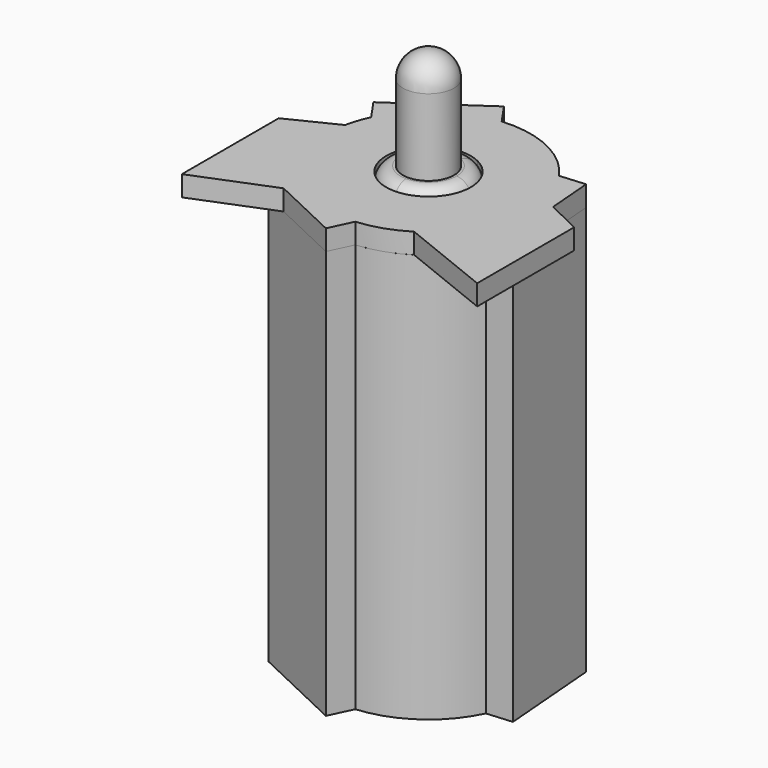
from build123d import *

# Parameters (mm, degrees)
F0_R     = 2.5
F1_DEPTH = 40
F2_DEPTH = 40
F3_R     = 2.5
F4_DEPTH = 10
F5_DEPTH = 2.5
F8_R     = 1.4
F9_DEPTH = 2


with BuildPart() as f1:
    # F0 (on Top) → F1 (new body)
    with BuildSketch(Plane.XY):
        with BuildLine():
            ThreePointArc((9.0374170739, -4.2807817782), (9.7563869014, -2.1938355979), (10, 0))
            ThreePointArc((10, 0), (9.5461967047, 2.9782760912), (8.2259743049, 5.6862418815))
            ThreePointArc((8.2259743049, 5.6862418815), (4.2807817782, 9.0374170739), (-0.8114427689, 9.9670236597))
            Line((-0.8114427689, 9.9670236597), (-9.0374170739, 4.2807817782))
            ThreePointArc((-9.0374170739, 4.2807817782), (-9.9670236597, -0.8114427689), (-8.2259743049, -5.6862418815))
            ThreePointArc((-8.2259743049, -5.6862418815), (-4.2807817782, -9.0374170739), (0.8114427689, -9.9670236597))
            ThreePointArc((0.8114427689, -9.9670236597), (5.6862418815, -8.2259743049), (9.0374170739, -4.2807817782))
        make_face()
        Circle(F0_R, mode=Mode.SUBTRACT)
        with BuildLine():
            ThreePointArc((8.2259743049, 5.6862418815), (9.5461967047, 2.9782760912), (10, 0))
            ThreePointArc((10, 0), (9.7563869014, -2.1938355979), (9.0374170739, -4.2807817782))
            Line((9.0374170739, -4.2807817782), (11.5291729888, -4.077921086))
            Line((11.5291729888, -4.077921086), (10.7177302199, 5.8891025737))
            Line((10.7177302199, 5.8891025737), (8.2259743049, 5.6862418815))
        make_face()
        with BuildLine():
            Line((-9.0374170739, 4.2807817782), (-0.8114427689, 9.9670236597))
            ThreePointArc((-0.8114427689, 9.9670236597), (-5.6862418815, 8.2259743049), (-9.0374170739, 4.2807817782))
        make_face()
        with BuildLine():
            ThreePointArc((-9.0374170739, 4.2807817782), (-5.6862418815, 8.2259743049), (-0.8114427689, 9.9670236597))
            Line((-0.8114427689, 9.9670236597), (-2.2330032393, 12.0235172359))
            Line((-2.2330032393, 12.0235172359), (-10.4589775442, 6.3372753545))
            Line((-10.4589775442, 6.3372753545), (-9.0374170739, 4.2807817782))
        make_face()
        with BuildLine():
            Line((-0.2587526756, -12.2263779282), (0.8114427689, -9.9670236597))
            ThreePointArc((0.8114427689, -9.9670236597), (-4.2807817782, -9.0374170739), (-8.2259743049, -5.6862418815))
            Line((-8.2259743049, -5.6862418815), (-9.2961697495, -7.9455961499))
            Line((-9.2961697495, -7.9455961499), (-0.2587526756, -12.2263779282))
        make_face()
    extrude(amount=F1_DEPTH)


with BuildPart() as f2:
    # F0 (on Top) → F2 (new body)
    with BuildSketch(Plane.XY):
        Circle(F0_R)
    extrude(amount=F2_DEPTH)

    # F3 (on face) → F4 (join)
    with BuildSketch(Plane.XY.offset(40)):
        Circle(F3_R)
    extrude(amount=F4_DEPTH)

    # F3 (on face) → F5 (join)
    with BuildSketch(Plane.XY.offset(40)):
        with BuildLine():
            ThreePointArc((1.8260342345, 3.7172857004), (-2.93e-08, 4.1415714414), (-1.8260342871, 3.7172856746))
            ThreePointArc((-1.8260342871, 3.7172856746), (-4.0341057369, -0.9373392702), (0, -4.1415714414))
            ThreePointArc((0, -4.1415714414), (2.928533251, -2.928533251), (4.1415714414, 0))
            ThreePointArc((4.1415714414, 0), (3.5153424613, 2.1897445933), (1.8260342345, 3.7172857004))
        make_face()
        Circle(F3_R, mode=Mode.SUBTRACT)
    extrude(amount=F5_DEPTH)

    # F6 (on Front) → F7 (revolve)
    with BuildSketch(Plane.XZ):
        with BuildLine():
            Line((-2.5, 50), (2.5, 50))
            ThreePointArc((2.5, 50), (0, 52.5), (-2.5, 50))
        make_face()
    revolve(axis=Axis((0, 0, 50), (-1, 0, 0)))

    # F8
    f8_edges = [f2.edges().sort_by_distance(p)[0] for p in [
        (1.826034, -3.717286, 42.5),
    ]]
    fillet(f8_edges, radius=F8_R)


with BuildPart() as f9:
    # F3 (on face) → F9 (new body)
    with BuildSketch(Plane.XY.offset(40)):
        with BuildLine():
            Line((11.2723216959, -0.9229938236), (1.8260342345, 3.7172857004))
            ThreePointArc((1.8260342345, 3.7172857004), (3.5153424613, 2.1897445933), (4.1415714414, 0))
            ThreePointArc((4.1415714414, 0), (2.928533251, -2.928533251), (0, -4.1415714414))
            Line((0, -4.1415714414), (7.1333343578, -7.008248065))
            ThreePointArc((7.1333343578, -7.008248065), (8.1995773399, -5.7242406874), (9.0374170739, -4.2807817782))
            Line((9.0374170739, -4.2807817782), (11.5291729888, -4.077921086))
            Line((11.5291729888, -4.077921086), (11.2723216959, -0.9229938236))
        make_face()
        with BuildLine():
            Line((1.8260342345, 3.7172857004), (0, 4.6142845799))
            Line((0, 4.6142845799), (-1.8260342871, 3.7172856746))
            ThreePointArc((-1.8260342871, 3.7172856746), (-2.93e-08, 4.1415714414), (1.8260342345, 3.7172857004))
        make_face()
        with BuildLine():
            ThreePointArc((-8.2259743049, -5.6862418815), (-9.5010919758, -3.1191747736), (-9.9956228645, -0.2958437956))
            Line((-9.9956228645, -0.2958437956), (-14.4493776544, -2.4836522061))
            Line((-14.4493776544, -2.4836522061), (-14.4493776544, -9.9483500207))
            Line((-14.4493776544, -9.9483500207), (-9.2562886562, -7.861400764))
            Line((-9.2562886562, -7.861400764), (-8.2259743049, -5.6862418815))
        make_face()
        with BuildLine():
            ThreePointArc((0, -4.1415714414), (-4.0341057369, -0.9373392702), (-1.8260342871, 3.7172856746))
            Line((-1.8260342871, 3.7172856746), (-9.9956228645, -0.2958437956))
            ThreePointArc((-9.9956228645, -0.2958437956), (-9.5010919758, -3.1191747736), (-8.2259743049, -5.6862418815))
            Line((-8.2259743049, -5.6862418815), (-9.2562886562, -7.861400764))
            Line((-9.2562886562, -7.861400764), (0, -4.1415714414))
        make_face()
        with BuildLine():
            Line((14.4493776544, -2.4836522061), (11.2723216959, -0.9229938236))
            Line((11.2723216959, -0.9229938236), (11.5291729888, -4.077921086))
            Line((11.5291729888, -4.077921086), (9.0374170739, -4.2807817782))
            ThreePointArc((9.0374170739, -4.2807817782), (8.1995773399, -5.7242406874), (7.1333343578, -7.008248065))
            Line((7.1333343578, -7.008248065), (14.4493776544, -9.9483500207))
            Line((14.4493776544, -9.9483500207), (14.4493776544, -2.4836522061))
        make_face()
        with BuildLine():
            Line((-14.4493776544, -2.4836522061), (-9.9956228645, -0.2958437956))
            ThreePointArc((-9.9956228645, -0.2958437956), (-9.9616891791, 0.8744991134), (-9.7911952771, 2.0328539162))
            Line((-9.7911952771, 2.0328539162), (-14.4493776544, -0.2553750195))
            Line((-14.4493776544, -0.2553750195), (-14.4493776544, -2.4836522061))
        make_face()
        Polygon((11.0833543073, 1.398109408), (11.2723216959, -0.9229938236), (14.4493776544, -2.4836522061), (14.4493776544, -0.2553750195), align=None)
        with BuildLine():
            Line((14.4493776544, -9.9483500207), (7.1333343578, -7.008248065))
            ThreePointArc((7.1333343578, -7.008248065), (6.2837328899, -7.7791195497), (5.3514333814, -8.4476127258))
            Line((5.3514333814, -8.4476127258), (14.4493776544, -12.1038081124))
            Line((14.4493776544, -12.1038081124), (14.4493776544, -9.9483500207))
        make_face()
        Polygon((-9.2961697495, -7.9455961499), (-9.2562886562, -7.861400764), (-14.4493776544, -9.9483500207), (-14.4493776544, -12.1038081124), (-6.9121769502, -9.0748295195), align=None)
        with BuildLine():
            Line((-1.8260342871, 3.7172856746), (0, 4.6142845799))
            Line((0, 4.6142845799), (1.8260342345, 3.7172857004))
            Line((1.8260342345, 3.7172857004), (11.2723216959, -0.9229938236))
            Line((11.2723216959, -0.9229938236), (11.0833543073, 1.398109408))
            Line((11.0833543073, 1.398109408), (0, 6.8425617666))
            Line((0, 6.8425617666), (-9.7911952771, 2.0328539162))
            ThreePointArc((-9.7911952771, 2.0328539162), (-9.9616891791, 0.8744991134), (-9.9956228645, -0.2958437956))
            Line((-9.9956228645, -0.2958437956), (-1.8260342871, 3.7172856746))
        make_face()
        with BuildLine():
            Line((7.1333343578, -7.008248065), (0, -4.1415714414))
            Line((0, -4.1415714414), (-9.2562886562, -7.861400764))
            Line((-9.2562886562, -7.861400764), (-9.2961697495, -7.9455961499))
            Line((-9.2961697495, -7.9455961499), (-6.9121769502, -9.0748295195))
            Line((-6.9121769502, -9.0748295195), (-0.2587526756, -12.2263779282))
            Line((-0.2587526756, -12.2263779282), (0.8114427689, -9.9670236597))
            ThreePointArc((0.8114427689, -9.9670236597), (3.1737065093, -9.4830157119), (5.3514333814, -8.4476127258))
            ThreePointArc((5.3514333814, -8.4476127258), (6.2837328899, -7.7791195497), (7.1333343578, -7.008248065))
        make_face()
        with BuildLine():
            ThreePointArc((-9.0374170739, 4.2807817782), (-9.4811632031, 3.1792364359), (-9.7911952771, 2.0328539162))
            Line((-9.7911952771, 2.0328539162), (0, 6.8425617666))
            Line((0, 6.8425617666), (11.0833543073, 1.398109408))
            Line((11.0833543073, 1.398109408), (10.7177302199, 5.8891025737))
            Line((10.7177302199, 5.8891025737), (8.2259743049, 5.6862418815))
            ThreePointArc((8.2259743049, 5.6862418815), (4.2807817782, 9.0374170739), (-0.8114427689, 9.9670236597))
            Line((-0.8114427689, 9.9670236597), (-2.2330032393, 12.0235172359))
            Line((-2.2330032393, 12.0235172359), (-10.4589775442, 6.3372753545))
            Line((-10.4589775442, 6.3372753545), (-9.0374170739, 4.2807817782))
        make_face()
    extrude(amount=F9_DEPTH)


solid = Compound([f1.part, f2.part, f9.part])
